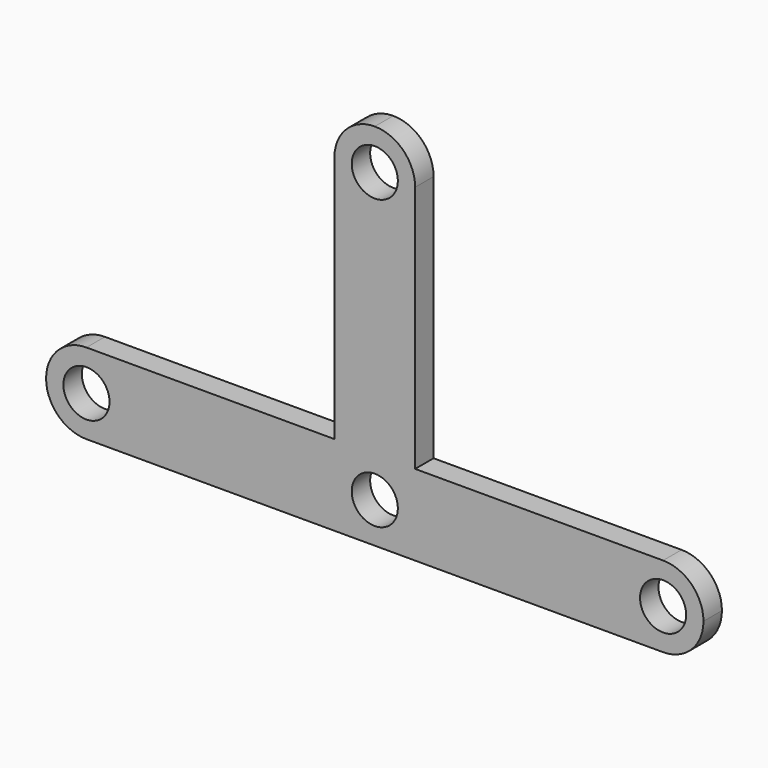
from build123d import *

# Parameters (mm, degrees)
F0_R     = 4
F1_DEPTH = 4
F2_R     = 6.99999


# Not quite as in the source:
# - a fillet or chamfer is up to 0.001 mm smaller than in the source, because OpenCascade refuses the exact size
# - a feature names something its author has since deleted; it is built from what else it names


with BuildPart() as f1:
    # F0 (on Front) → F1 (new body)
    with BuildSketch(Plane.XZ):
        Polygon((7, 57), (-7, 57), (-7, 7), (-57, 7), (-57, -7), (57, -7), (57, 7), (7, 7), align=None)
        with Locations((-50, 0)):
            Circle(F0_R, mode=Mode.SUBTRACT)
        Circle(F0_R, mode=Mode.SUBTRACT)
        with Locations((50, 0)):
            Circle(F0_R, mode=Mode.SUBTRACT)
        with Locations((0, 50)):
            Circle(F0_R, mode=Mode.SUBTRACT)
    extrude(amount=F1_DEPTH)

    # F2 (radius 7 in the source; OpenCascade refuses exactly that, so slightly less here)
    f2_edges = [f1.edges().sort_by_distance(p)[0] for p in [
        (57, -2, -7),
        (57, -2, 7),
        (7, -2, 57),
        (-7, -2, 57),
        (-57, -2, 7),
        (-57, -2, -7),
    ]]
    fillet(f2_edges, radius=F2_R)


solid = f1.part
